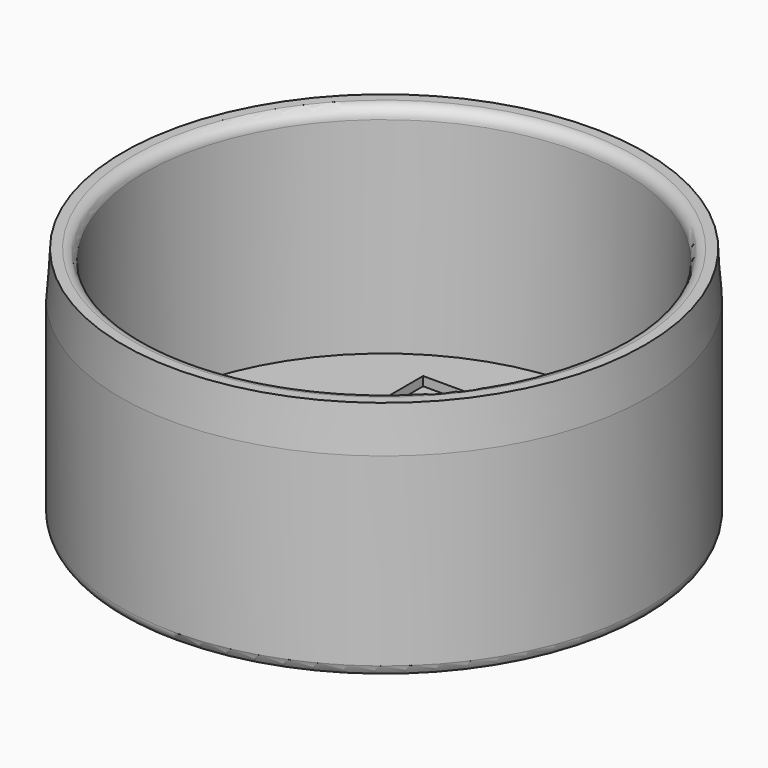
from build123d import *

# Parameters (mm, degrees)
F0_R         = 15.9
F1_DEPTH     = 1.6
F0_R_2       = 17.5
F2_DEPTH     = 16
F3_SIZE2     = 3
F3_SIZE      = 0.2
F4_R         = 0.75
F0_TEXT_SIZE = 32.465683762
F5_DEPTH     = 1
F6_DEPTH     = 1.6


# Not quite as in the source:
# - Text() gives the source's letters only with a copy of the font that has no kerning and outlines rounded to 1/6400 em; it was checked with that copy


with BuildPart() as f1:
    # F0 (on Top) → F1 (new body)
    with BuildSketch(Plane.XY):
        Circle(F0_R)
        with BuildLine():
            Line((-6.777657014, -11.4727395121), (-6.777657014, 11.7047150361))
            Line((-6.777657014, 11.7047150361), (-0.2287198677, 11.7047150361))
            add(Edge.make_bspline(
                [(-0.2287198677, 11.7047150361), (4.3824217792, 11.7047150361), (6.4444999744, 10.3249234762)],
                knots=[0, 0, 0, 1, 1, 1], degree=2))
            add(Edge.make_bspline(
                [(6.4444999744, 10.3249234762), (8.5065781695, 8.9451319163), (8.5065781695, 5.9674199838)],
                knots=[0, 0, 0, 1, 1, 1], degree=2))
            add(Edge.make_bspline(
                [(8.5065781695, 5.9674199838), (8.5065781695, 3.9028054071), (7.3575973302, 2.5635959519)],
                knots=[0, 0, 0, 1, 1, 1], degree=2))
            add(Edge.make_bspline(
                [(7.3575973302, 2.5635959519), (6.2086164908, 1.2243864967), (4.0019645476, 0.8287109758)],
                knots=[0, 0, 0, 1, 1, 1], degree=2))
            Line((4.0019645476, 0.8287109758), (4.0019645476, 0.6714553201))
            add(Edge.make_bspline(
                [(4.0019645476, 0.6714553201), (9.282710922, -0.2314965095), (9.282710922, -4.8781474979)],
                knots=[0, 0, 0, 1, 1, 1], degree=2))
            add(Edge.make_bspline(
                [(9.282710922, -4.8781474979), (9.282710922, -7.9826785077), (7.1825870036, -9.7277090099)],
                knots=[0, 0, 0, 1, 1, 1], degree=2))
            add(Edge.make_bspline(
                [(7.1825870036, -9.7277090099), (5.0824630853, -11.4727395121), (1.3083273479, -11.4727395121)],
                knots=[0, 0, 0, 1, 1, 1], degree=2))
            Line((1.3083273479, -11.4727395121), (-6.777657014, -11.4727395121))
        make_face(mode=Mode.SUBTRACT)
    extrude(amount=F1_DEPTH)

    # F0 (on Top) → F2 (join)
    with BuildSketch(Plane.XY):
        Circle(F0_R_2)
        Circle(F0_R, mode=Mode.SUBTRACT)
    extrude(amount=F2_DEPTH)

    # F3
    f3_edges = [f1.edges().sort_by_distance(p)[0] for p in [
        (-17.5, 0, 16),
    ]]
    f3_side = f1.faces().sort_by_distance((-17.005025, 0, 16))[0]
    chamfer(f3_edges, length=F3_SIZE, length2=F3_SIZE2, reference=f3_side)

    # F4
    f4_edges = [f1.edges().sort_by_distance(p)[0] for p in [
        (-17.5, 0, 0),
        (-15.9, 0, 16),
    ]]
    fillet(f4_edges, radius=F4_R)

    # F0 (on Top) → F5 (join)
    with BuildSketch(Plane.XY):
        with Locations((-9.9633522332, -11.4727395121)):
            Text('B', F0_TEXT_SIZE, font='Open Sans', text_align=(TextAlign.LEFT, TextAlign.BOTTOM))
    extrude(amount=F5_DEPTH)

    # F0 (on Top) → F6 (join)
    with BuildSketch(Plane.XY):
        with BuildLine():
            Line((-4.0840198144, 9.3712440157), (-4.0840198144, 1.7823904363))
            Line((-4.0840198144, 1.7823904363), (0.3546478874, 1.7823904363))
            add(Edge.make_bspline(
                [(0.3546478874, 1.7823904363), (3.2106135059, 1.7823904363), (4.4635859886, 2.6777331213)],
                knots=[0, 0, 0, 1, 1, 1], degree=2))
            add(Edge.make_bspline(
                [(4.4635859886, 2.6777331213), (5.7165584712, 3.5730758063), (5.7165584712, 5.693490777)],
                knots=[0, 0, 0, 1, 1, 1], degree=2))
            add(Edge.make_bspline(
                [(5.7165584712, 5.693490777), (5.7165584712, 7.6465045659), (4.3215486221, 8.5088742908)],
                knots=[0, 0, 0, 1, 1, 1], degree=2))
            add(Edge.make_bspline(
                [(4.3215486221, 8.5088742908), (2.926538773, 9.3712440157), (-0.1171190797, 9.3712440157)],
                knots=[0, 0, 0, 1, 1, 1], degree=2))
            Line((-0.1171190797, 9.3712440157), (-4.0840198144, 9.3712440157))
        make_face()
        with BuildLine():
            Line((0.5321945955, -0.5003529532), (-4.0840198144, -0.5003529532))
            Line((-4.0840198144, -0.5003529532), (-4.0840198144, -9.1747778333))
            Line((-4.0840198144, -9.1747778333), (0.7553961714, -9.1747778333))
            add(Edge.make_bspline(
                [(0.7553961714, -9.1747778333), (3.5606341589, -9.1747778333), (4.978471442, -8.0892065325)],
                knots=[0, 0, 0, 1, 1, 1], degree=2))
            add(Edge.make_bspline(
                [(4.978471442, -8.0892065325), (6.396308725, -7.0036352317), (6.396308725, -4.6853825006)],
                knots=[0, 0, 0, 1, 1, 1], degree=2))
            add(Edge.make_bspline(
                [(6.396308725, -4.6853825006), (6.396308725, -2.5294581883), (4.9454984819, -1.5149055707)],
                knots=[0, 0, 0, 1, 1, 1], degree=2))
            add(Edge.make_bspline(
                [(4.9454984819, -1.5149055707), (3.4946882388, -0.5003529532), (0.5321945955, -0.5003529532)],
                knots=[0, 0, 0, 1, 1, 1], degree=2))
        make_face()
    extrude(amount=F6_DEPTH)


solid = f1.part
